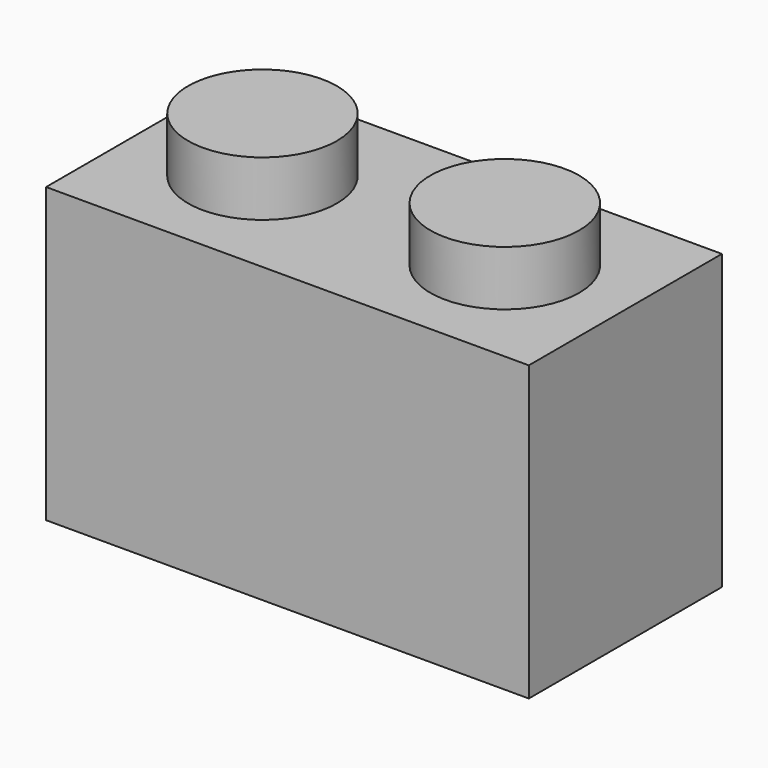
from build123d import *

# Parameters (mm, degrees)
F0_W     = 15.8
F0_H     = 7.9
F0_R     = 2.435
F1_DEPTH = 9.6
F2_DEPTH = 11.4
F3_T     = -1.4


# Not quite as in the source:
# - a feature names something its author has since deleted; it is built from what else it names


with BuildPart() as f1:
    # F0 (on Top) → F1 (new body)
    with BuildSketch(Plane.XY):
        with Locations((0, -3.95)):
            Rectangle(F0_W, F0_H)
        with Locations((-3.965, -3.965)):
            Circle(F0_R, mode=Mode.SUBTRACT)
        with Locations((3.965, -3.965)):
            Circle(F0_R, mode=Mode.SUBTRACT)
    extrude(amount=F1_DEPTH)

    # F0 (on Top) → F2 (join)
    with BuildSketch(Plane.XY):
        with Locations((3.965, -3.965)):
            Circle(F0_R)
        with Locations((-3.965, -3.965)):
            Circle(F0_R)
    extrude(amount=F2_DEPTH)

    # F3
    f3_openings = [f1.faces().sort_by_distance(p)[0] for p in [
        (0, -3.95, 0),
    ]]
    offset(amount=F3_T, openings=f3_openings, kind=Kind.INTERSECTION)


solid = f1.part
